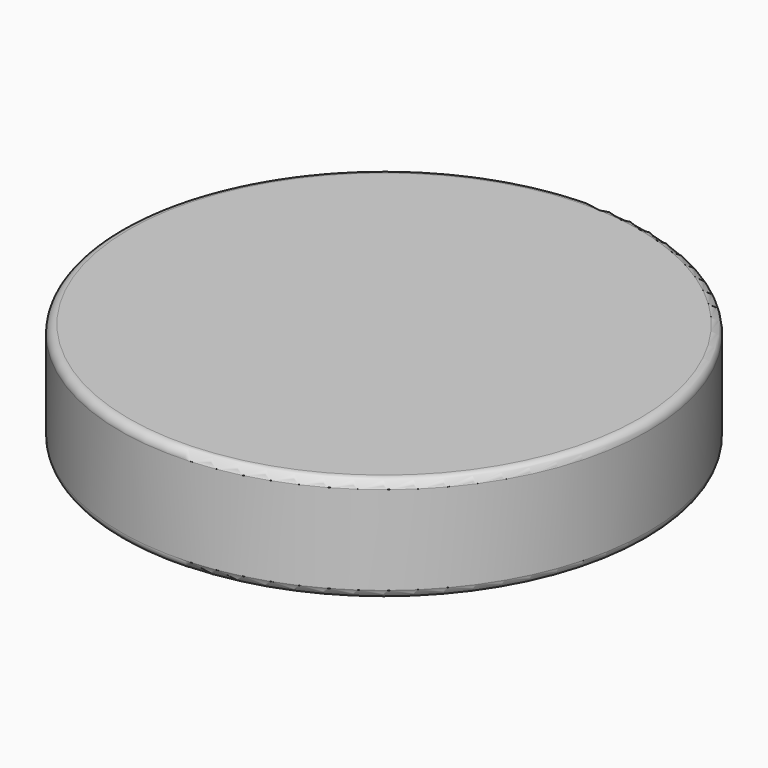
from build123d import *

# Parameters (mm, degrees)
F0_R     = 6.35
F1_DEPTH = 1.27
F2_R     = 0.2032
F3_R     = 5.207
F3_R_2   = 4.191
F3_R_3   = 2.54
F3_R_4   = 1.524
F4_DEPTH = 0.254
F5_R     = 0.2032


with BuildPart() as f1:
    # F0 (on Top) → F1 (new body, symmetric)
    with BuildSketch(Plane.XY):
        Circle(F0_R)
    extrude(amount=F1_DEPTH, both=True)

    # F2
    f2_edges = [f1.edges().sort_by_distance(p)[0] for p in [
        (-6.35, 0, -1.27),
        (-6.35, 0, 1.27),
    ]]
    fillet(f2_edges, radius=F2_R)

    # F3 (on face) → F4 (cut)
    with BuildSketch(Plane(origin=(0, 0, -1.27), x_dir=(1, 0, 0), z_dir=(0, 0, -1))):
        Circle(F3_R)
        Circle(F3_R_2, mode=Mode.SUBTRACT)
        Circle(F3_R_3)
        Circle(F3_R_4, mode=Mode.SUBTRACT)
    extrude(amount=-F4_DEPTH, mode=Mode.SUBTRACT)

    # F5
    f5_edges = [f1.edges().sort_by_distance(p)[0] for p in [
        (-5.207, 0, -1.27),
        (-4.191, 0, -1.27),
        (-2.54, 0, -1.27),
        (-1.524, 0, -1.27),
    ]]
    fillet(f5_edges, radius=F5_R)


solid = f1.part
